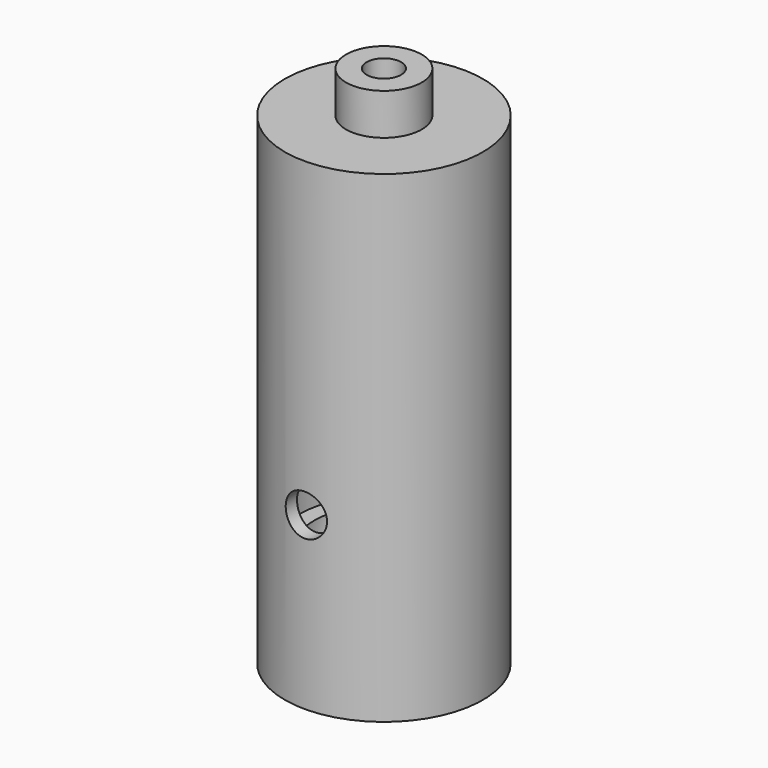
from build123d import *

# Parameters (mm, degrees)
F0_W     = 3
F0_H     = 6
F2_R     = 3
F3_DEPTH = 15


# Not quite as in the source:
# - a feature names something its author has since deleted; it is built from what else it names


with BuildPart() as f1:
    # F0 (on Front) → F1 (revolve)
    with BuildSketch(Plane.XZ):
        with BuildLine():
            Line((-5.5, 35), (-14.375, 35))
            Line((-14.375, 35), (-14.375, -35))
            Line((-14.375, -35), (0, -35))
            Line((0, -35), (0, -30.075))
            ThreePointArc((0, -30.075), (-7.1241008205, -27.1241008205), (-10.075, -20))
            Line((-10.075, -20), (-12.375, -20))
            Line((-12.375, -20), (-12.375, -0.2))
            Line((-12.375, -0.2), (-10.075, -0.2))
            Line((-10.075, -0.2), (-10.075, 20))
            ThreePointArc((-10.075, 20), (-7.9590553774, 26.1773022024), (-2.5, 29.7598988212))
            Line((-2.5, 29.7598988212), (-2.5, 35))
            Line((-2.5, 35), (-5.5, 35))
        make_face()
        with Locations((-4, 38)):
            Rectangle(F0_W, F0_H)
    revolve(axis=Axis((0, 0, 0), (0, 0, -1)))

    # F2 (on Front) → F3 (cut, symmetric)
    with BuildSketch(Plane.XZ):
        with Locations((0, -10.2)):
            Circle(F2_R)
    extrude(amount=F3_DEPTH, both=True, mode=Mode.SUBTRACT)


solid = f1.part
